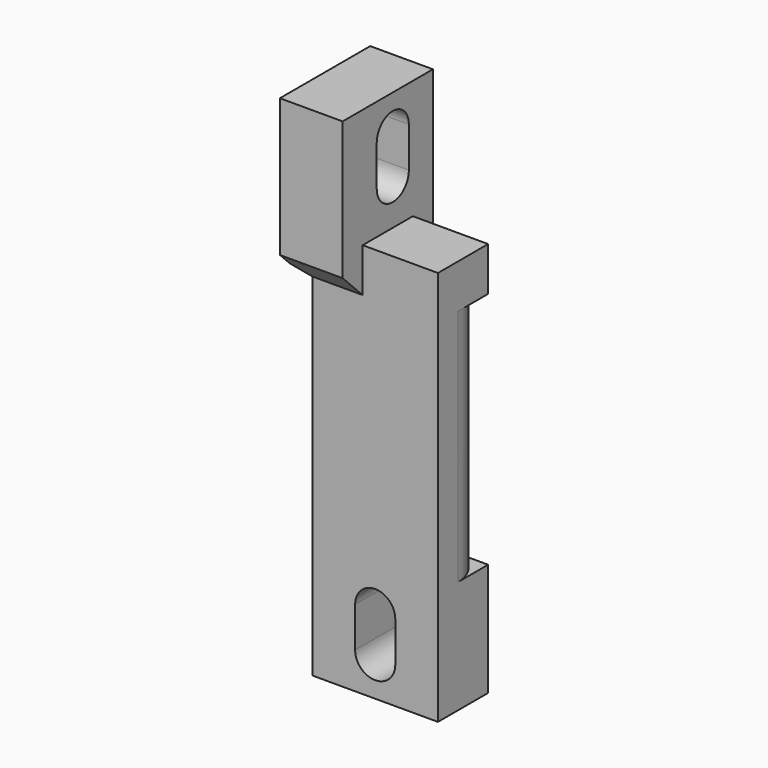
from build123d import *

# Parameters (mm, degrees)
F1_DEPTH      = 5
F4_DEPTH      = 2
F4_DEPTH_BACK = 7
F6_DEPTH      = 25
F7_SIZE       = 2
F8_SIZE       = 0.99999
F10_DEPTH     = 19
F11_SIZE      = 1


# Not quite as in the source:
# - a fillet or chamfer is up to 0.001 mm smaller than in the source, because OpenCascade refuses the exact size


with BuildPart() as f1:
    # F0 (on Front) → F1 (new body)
    with BuildSketch(Plane.XZ):
        Polygon((0, 28), (0, 0), (10, 0), (10, 31.5), (4, 31.5), (4, 41), (-1, 41), (-1, 28), align=None)
        with BuildLine():
            ThreePointArc((3.4, 6.1), (5, 7.7), (6.6, 6.1))
            Line((6.6, 6.1), (6.6, 2.9))
            ThreePointArc((6.6, 2.9), (5, 1.3), (3.4, 2.9))
            Line((3.4, 2.9), (3.4, 6.1))
        make_face(mode=Mode.SUBTRACT)
    extrude(amount=F1_DEPTH)

    # F3 (on face) → F4 (join, two sides)
    with BuildSketch(Plane(origin=(0, 0, 0), x_dir=(-1, 0, 0), z_dir=(0, 1, 0))) as f4_sk:
        Polygon((1, 28), (1, 41), (-4, 41), (-4, 31.5), (-4, 28), (0, 28), align=None)
    extrude(amount=F4_DEPTH)
    extrude(f4_sk.sketch, amount=-F4_DEPTH_BACK)

    # F5 (on face) → F6 (cut)
    with BuildSketch(Plane(origin=(-1, 0, 0), x_dir=(0, -1, 0), z_dir=(-1, 0, 0))):
        with BuildLine():
            Line((3.6, 34.9), (3.6, 38.1))
            ThreePointArc((3.6, 38.1), (2, 39.7), (0.4, 38.1))
            Line((0.4, 38.1), (0.4, 34.9))
            ThreePointArc((0.4, 34.9), (2, 33.3), (3.6, 34.9))
        make_face()
    extrude(amount=-F6_DEPTH, mode=Mode.SUBTRACT)

    # F7
    f7_edges = [f1.edges().sort_by_distance(p)[0] for p in [
        (1.5, 2, 28),
        (1.5, -7, 28),
    ]]
    chamfer(f7_edges, length=F7_SIZE)

    # F8 (size 1 in the source; OpenCascade refuses exactly that, so slightly less here)
    f8_edges = [f1.edges().sort_by_distance(p)[0] for p in [
        (-1, -2.5, 28),
    ]]
    chamfer(f8_edges, length=F8_SIZE)

    # F9 (on offset) → F10 (cut)
    with BuildSketch(Plane.XY.offset(9)):
        with BuildLine():
            Line((10, 0), (7, 0))
            ThreePointArc((7, 0), (9.1213203436, -0.8786796564), (10, -3))
            Line((10, -3), (10, 0))
        make_face()
        with BuildLine():
            ThreePointArc((0, -3), (0.8786796564, -0.8786796564), (3, 0))
            Line((3, 0), (0, 0))
            Line((0, 0), (0, -3))
        make_face()
    extrude(amount=F10_DEPTH, mode=Mode.SUBTRACT)

    # F11
    f11_edges = [f1.edges().sort_by_distance(p)[0] for p in [
        (6.6, 0, 4.5),
        (-1, -3.6, 36.5),
    ]]
    chamfer(f11_edges, length=F11_SIZE)


solid = f1.part
